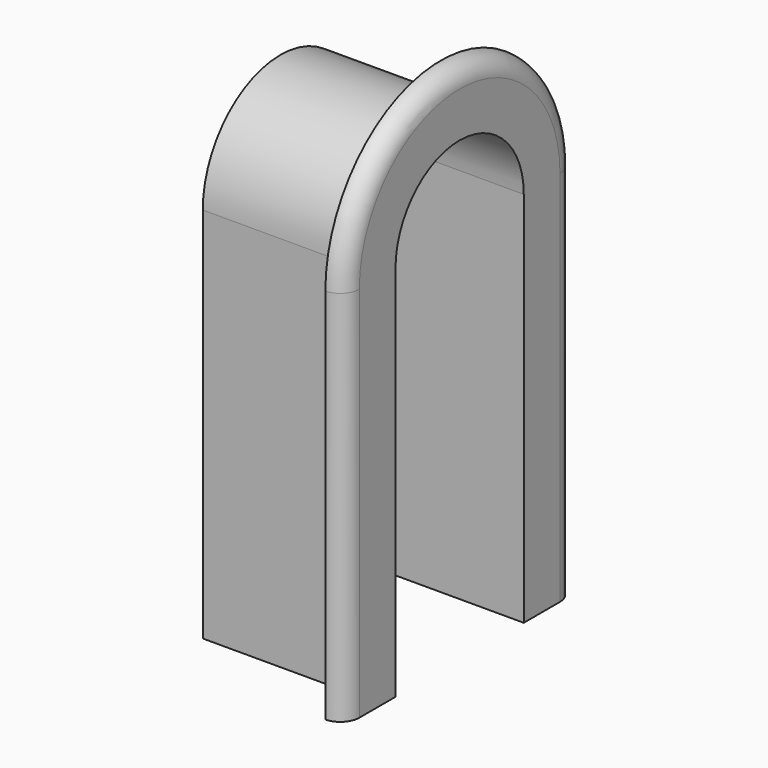
from build123d import *

# Parameters (mm, degrees)
F1_DEPTH = 17
F3_DEPTH = 2
F4_R     = 1.99999


# Not quite as in the source:
# - a fillet or chamfer is up to 0.001 mm smaller than in the source, because OpenCascade refuses the exact size
# - a feature of the source that left no trace in its solid (it failed there, or was rolled back) is left out


with BuildPart() as f1:
    # F0 (on Right) → F1 (new body)
    with BuildSketch(Plane.YZ):
        with BuildLine():
            Line((-1.8, 0), (0, 0))
            Line((0, 0), (0, 40))
            ThreePointArc((0, 40), (8.5, 48.5), (17, 40))
            Line((17, 40), (17, 0))
            Line((17, 0), (18.8, 0))
            Line((18.8, 0), (18.8, 40))
            ThreePointArc((18.8, 40), (8.5, 50.3), (-1.8, 40))
            Line((-1.8, 40), (-1.8, 0))
        make_face()
    extrude(amount=F1_DEPTH)

    # F2 (on face) → F3 (join)
    with BuildSketch(Plane.YZ.offset(17)):
        with BuildLine():
            ThreePointArc((-1.8, 40), (8.5, 50.3), (18.8, 40))
            Line((18.8, 40), (18.8, 0))
            Line((18.8, 0), (23.8, 0))
            Line((23.8, 0), (23.8, 40))
            ThreePointArc((23.8, 40), (8.5, 55.3), (-6.8, 40))
            Line((-6.8, 40), (-6.8, 0))
            Line((-6.8, 0), (-1.8, 0))
            Line((-1.8, 0), (-1.8, 40))
        make_face()
        with BuildLine():
            Line((18.8, 0), (18.8, 40))
            ThreePointArc((18.8, 40), (8.5, 50.3), (-1.8, 40))
            Line((-1.8, 40), (-1.8, 0))
            Line((-1.8, 0), (0, 0))
            Line((0, 0), (0, 40))
            ThreePointArc((0, 40), (8.5, 48.5), (17, 40))
            Line((17, 40), (17, 0))
            Line((17, 0), (18.8, 0))
        make_face()
    extrude(amount=F3_DEPTH)

    # F4 (radius 2 in the source; OpenCascade refuses exactly that, so slightly less here)
    f4_edges = [f1.edges().sort_by_distance(p)[0] for p in [
        (19, -6.8, 20),
        (19, 8.5, 55.3),
        (19, 23.8, 20),
    ]]
    fillet(f4_edges, radius=F4_R)


solid = f1.part
